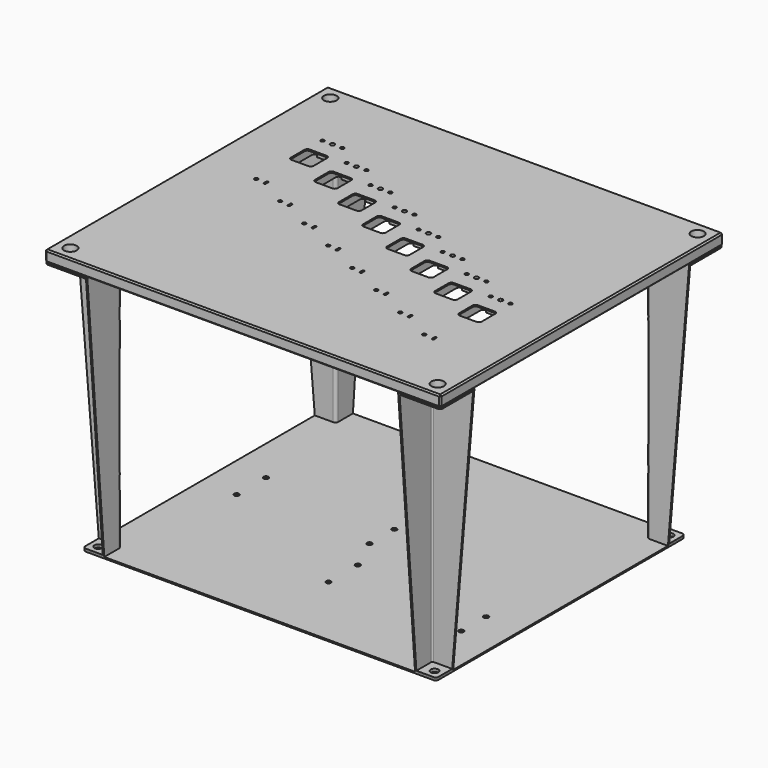
from build123d import *

# Parameters (mm, degrees)
F0_W              = 280
F0_H              = 250
F0_R              = 1.25
F0_R_2            = 1.525
F1_DEPTH          = 8
F2_W              = 30
F2_H              = 30
F4_W              = 15
F4_H              = 15
F9_T              = -1
F9_2_T            = -1
F9_3_T            = -1
F9_4_T            = -1
F10_W             = 250
F10_H             = 220
F11_DEPTH         = 1
F12_R             = 2.75
F13_DEPTH         = 25
F15_D             = 5.5
F15_DEPTH         = 20
F15_CBORE_D       = 9
F15_CBORE_DEPTH   = 5.5
F15_TIP           = 1.6523667023
F15_2_D           = 5.5
F15_2_DEPTH       = 20
F15_2_CBORE_D     = 9
F15_2_CBORE_DEPTH = 5.5
F15_2_TIP         = 1.6523667023
F15_3_D           = 5.5
F15_3_DEPTH       = 20
F15_3_CBORE_D     = 9
F15_3_CBORE_DEPTH = 5.5
F15_3_TIP         = 1.6523667023
F15_4_D           = 5.5
F15_4_DEPTH       = 20
F15_4_CBORE_D     = 9
F15_4_CBORE_DEPTH = 5.5
F15_4_TIP         = 1.6523667023
F15_5_D           = 5.5
F15_5_DEPTH       = 20
F15_5_CBORE_D     = 9
F15_5_CBORE_DEPTH = 5.5
F15_5_TIP         = 1.6523667023
F16_R             = 2
F16_2_R           = 2
F16_3_R           = 2
F16_4_R           = 2
F17_R             = 1
F17_2_R           = 1
F17_3_R           = 1
F17_4_R           = 1
F19_DEPTH         = 7
F21_DEPTH         = 5
F22_R             = 1.75
F23_DEPTH         = 1.001
F24_SIZE          = 1
F25_R             = 2
F25_2_R           = 2
F25_3_R           = 2
F25_4_R           = 2
F25_5_R           = 2


with BuildPart() as f1:
    # F0 (on Top) → F1 (new body)
    with BuildSketch(Plane.XY):
        Rectangle(F0_W, F0_H)
        with Locations((-47.5, -11.22)):
            Circle(F0_R, mode=Mode.SUBTRACT)
        with BuildLine():
            Line((-41.265, -12.22), (-41.265, -10.22))
            ThreePointArc((-41.265, -10.22), (-40.5, -9.455), (-39.735, -10.22))
            Line((-39.735, -10.22), (-39.735, -12.22))
            ThreePointArc((-39.735, -12.22), (-40.5, -12.985), (-41.265, -12.22))
        make_face(mode=Mode.SUBTRACT)
        with Locations((-20.5, -23.72)):
            Circle(F0_R, mode=Mode.SUBTRACT)
        with BuildLine():
            Line((-12.735, -22.72), (-12.735, -24.72))
            ThreePointArc((-12.735, -24.72), (-13.5, -25.485), (-14.265, -24.72))
            Line((-14.265, -24.72), (-14.265, -22.72))
            ThreePointArc((-14.265, -22.72), (-13.5, -21.955), (-12.735, -22.72))
        make_face(mode=Mode.SUBTRACT)
        with Locations((87.5, -73.72)):
            Circle(F0_R, mode=Mode.SUBTRACT)
        with BuildLine():
            Line((95.265, -72.72), (95.265, -74.72))
            ThreePointArc((95.265, -74.72), (94.5, -75.485), (93.735, -74.72))
            Line((93.735, -74.72), (93.735, -72.72))
            ThreePointArc((93.735, -72.72), (94.5, -71.955), (95.265, -72.72))
        make_face(mode=Mode.SUBTRACT)
        with Locations((33.5, -48.72)):
            Circle(F0_R, mode=Mode.SUBTRACT)
        with Locations((6.5, -36.22)):
            Circle(F0_R, mode=Mode.SUBTRACT)
        with BuildLine():
            Line((14.265, -35.22), (14.265, -37.22))
            ThreePointArc((14.265, -37.22), (13.5, -37.985), (12.735, -37.22))
            Line((12.735, -37.22), (12.735, -35.22))
            ThreePointArc((12.735, -35.22), (13.5, -34.455), (14.265, -35.22))
        make_face(mode=Mode.SUBTRACT)
        with BuildLine():
            Line((41.265, -47.72), (41.265, -49.72))
            ThreePointArc((41.265, -49.72), (40.5, -50.485), (39.735, -49.72))
            Line((39.735, -49.72), (39.735, -47.72))
            ThreePointArc((39.735, -47.72), (40.5, -46.955), (41.265, -47.72))
        make_face(mode=Mode.SUBTRACT)
        with Locations((60.5, -61.22)):
            Circle(F0_R, mode=Mode.SUBTRACT)
        with BuildLine():
            Line((68.265, -60.22), (68.265, -62.22))
            ThreePointArc((68.265, -62.22), (67.5, -62.985), (66.735, -62.22))
            Line((66.735, -62.22), (66.735, -60.22))
            ThreePointArc((66.735, -60.22), (67.5, -59.455), (68.265, -60.22))
        make_face(mode=Mode.SUBTRACT)
        with BuildLine():
            Line((73.5, -31.2), (61.5, -31.2))
            ThreePointArc((61.5, -31.2), (60.0857864376, -30.6142135624), (59.5, -29.2))
            Line((59.5, -29.2), (59.5, -17.2))
            ThreePointArc((59.5, -17.2), (60.0857864376, -15.7857864376), (61.5, -15.2))
            Line((61.5, -15.2), (73.5, -15.2))
            ThreePointArc((73.5, -15.2), (74.9142135624, -15.7857864376), (75.5, -17.2))
            Line((75.5, -17.2), (75.5, -29.2))
            ThreePointArc((75.5, -29.2), (74.9142135624, -30.6142135624), (73.5, -31.2))
        make_face(mode=Mode.SUBTRACT)
        with BuildLine():
            Line((46.5, -18.7), (34.5, -18.7))
            ThreePointArc((34.5, -18.7), (33.0857864376, -18.1142135624), (32.5, -16.7))
            Line((32.5, -16.7), (32.5, -4.7))
            ThreePointArc((32.5, -4.7), (33.0857864376, -3.2857864376), (34.5, -2.7))
            Line((34.5, -2.7), (46.5, -2.7))
            ThreePointArc((46.5, -2.7), (47.9142135624, -3.2857864376), (48.5, -4.7))
            Line((48.5, -4.7), (48.5, -16.7))
            ThreePointArc((48.5, -16.7), (47.9142135624, -18.1142135624), (46.5, -18.7))
        make_face(mode=Mode.SUBTRACT)
        with Locations((60.5, -2.5)):
            Circle(F0_R, mode=Mode.SUBTRACT)
        with Locations((67.5, -2.5)):
            Circle(F0_R_2, mode=Mode.SUBTRACT)
        with BuildLine():
            Line((100.5, -43.7), (88.5, -43.7))
            ThreePointArc((88.5, -43.7), (87.0857864376, -43.1142135624), (86.5, -41.7))
            Line((86.5, -41.7), (86.5, -29.7))
            ThreePointArc((86.5, -29.7), (87.0857864376, -28.2857864376), (88.5, -27.7))
            Line((88.5, -27.7), (100.5, -27.7))
            ThreePointArc((100.5, -27.7), (101.9142135624, -28.2857864376), (102.5, -29.7))
            Line((102.5, -29.7), (102.5, -41.7))
            ThreePointArc((102.5, -41.7), (101.9142135624, -43.1142135624), (100.5, -43.7))
        make_face(mode=Mode.SUBTRACT)
        with Locations((74.5, -2.5)):
            Circle(F0_R, mode=Mode.SUBTRACT)
        with Locations((87.5, -15)):
            Circle(F0_R, mode=Mode.SUBTRACT)
        with Locations((94.5, -15)):
            Circle(F0_R_2, mode=Mode.SUBTRACT)
        with Locations((101.5, -15)):
            Circle(F0_R, mode=Mode.SUBTRACT)
        with Locations((-101.5, 13.78)):
            Circle(F0_R, mode=Mode.SUBTRACT)
        with BuildLine():
            Line((-93.735, 14.78), (-93.735, 12.78))
            ThreePointArc((-93.735, 12.78), (-94.5, 12.015), (-95.265, 12.78))
            Line((-95.265, 12.78), (-95.265, 14.78))
            ThreePointArc((-95.265, 14.78), (-94.5, 15.545), (-93.735, 14.78))
        make_face(mode=Mode.SUBTRACT)
        with Locations((-74.5, 1.28)):
            Circle(F0_R, mode=Mode.SUBTRACT)
        with BuildLine():
            Line((-88.5, 43.8), (-100.5, 43.8))
            ThreePointArc((-100.5, 43.8), (-101.9142135624, 44.3857864376), (-102.5, 45.8))
            Line((-102.5, 45.8), (-102.5, 57.8))
            ThreePointArc((-102.5, 57.8), (-101.9142135624, 59.2142135624), (-100.5, 59.8))
            Line((-100.5, 59.8), (-88.5, 59.8))
            ThreePointArc((-88.5, 59.8), (-87.0857864376, 59.2142135624), (-86.5, 57.8))
            Line((-86.5, 57.8), (-86.5, 45.8))
            ThreePointArc((-86.5, 45.8), (-87.0857864376, 44.3857864376), (-88.5, 43.8))
        make_face(mode=Mode.SUBTRACT)
        with Locations((-74.5, 60)):
            Circle(F0_R, mode=Mode.SUBTRACT)
        with BuildLine():
            Line((-66.735, 2.28), (-66.735, 0.28))
            ThreePointArc((-66.735, 0.28), (-67.5, -0.485), (-68.265, 0.28))
            Line((-68.265, 0.28), (-68.265, 2.28))
            ThreePointArc((-68.265, 2.28), (-67.5, 3.045), (-66.735, 2.28))
        make_face(mode=Mode.SUBTRACT)
        with BuildLine():
            ThreePointArc((-48.5, 32.8), (-47.9142135624, 34.2142135624), (-46.5, 34.8))
            Line((-46.5, 34.8), (-34.5, 34.8))
            ThreePointArc((-34.5, 34.8), (-33.0857864376, 34.2142135624), (-32.5, 32.8))
            Line((-32.5, 32.8), (-32.5, 20.8))
            ThreePointArc((-32.5, 20.8), (-33.0857864376, 19.3857864376), (-34.5, 18.8))
            Line((-34.5, 18.8), (-46.5, 18.8))
            ThreePointArc((-46.5, 18.8), (-47.9142135624, 19.3857864376), (-48.5, 20.8))
            Line((-48.5, 20.8), (-48.5, 32.8))
        make_face(mode=Mode.SUBTRACT)
        with BuildLine():
            Line((-7.5, 6.3), (-19.5, 6.3))
            ThreePointArc((-19.5, 6.3), (-20.9142135624, 6.8857864376), (-21.5, 8.3))
            Line((-21.5, 8.3), (-21.5, 20.3))
            ThreePointArc((-21.5, 20.3), (-20.9142135624, 21.7142135624), (-19.5, 22.3))
            Line((-19.5, 22.3), (-7.5, 22.3))
            ThreePointArc((-7.5, 22.3), (-6.0857864376, 21.7142135624), (-5.5, 20.3))
            Line((-5.5, 20.3), (-5.5, 8.3))
            ThreePointArc((-5.5, 8.3), (-6.0857864376, 6.8857864376), (-7.5, 6.3))
        make_face(mode=Mode.SUBTRACT)
        with BuildLine():
            Line((-61.5, 31.3), (-73.5, 31.3))
            ThreePointArc((-73.5, 31.3), (-74.9142135624, 31.8857864376), (-75.5, 33.3))
            Line((-75.5, 33.3), (-75.5, 45.3))
            ThreePointArc((-75.5, 45.3), (-74.9142135624, 46.7142135624), (-73.5, 47.3))
            Line((-73.5, 47.3), (-61.5, 47.3))
            ThreePointArc((-61.5, 47.3), (-60.0857864376, 46.7142135624), (-59.5, 45.3))
            Line((-59.5, 45.3), (-59.5, 33.3))
            ThreePointArc((-59.5, 33.3), (-60.0857864376, 31.8857864376), (-61.5, 31.3))
        make_face(mode=Mode.SUBTRACT)
        with Locations((-67.5, 60)):
            Circle(F0_R_2, mode=Mode.SUBTRACT)
        with Locations((-60.5, 60)):
            Circle(F0_R, mode=Mode.SUBTRACT)
        with Locations((-47.5, 47.5)):
            Circle(F0_R, mode=Mode.SUBTRACT)
        with Locations((-40.5, 47.5)):
            Circle(F0_R_2, mode=Mode.SUBTRACT)
        with Locations((-20.5, 35)):
            Circle(F0_R, mode=Mode.SUBTRACT)
        with Locations((-13.5, 35)):
            Circle(F0_R_2, mode=Mode.SUBTRACT)
        with Locations((-6.5, 35)):
            Circle(F0_R, mode=Mode.SUBTRACT)
        with Locations((-33.5, 47.5)):
            Circle(F0_R, mode=Mode.SUBTRACT)
        with Locations((-101.5, 72.5)):
            Circle(F0_R, mode=Mode.SUBTRACT)
        with Locations((-94.5, 72.5)):
            Circle(F0_R_2, mode=Mode.SUBTRACT)
        with Locations((-87.5, 72.5)):
            Circle(F0_R, mode=Mode.SUBTRACT)
        with BuildLine():
            Line((19.5, -6.2), (7.5, -6.2))
            ThreePointArc((7.5, -6.2), (6.0857864376, -5.6142135624), (5.5, -4.2))
            Line((5.5, -4.2), (5.5, 7.8))
            ThreePointArc((5.5, 7.8), (6.0857864376, 9.2142135624), (7.5, 9.8))
            Line((7.5, 9.8), (19.5, 9.8))
            ThreePointArc((19.5, 9.8), (20.9142135624, 9.2142135624), (21.5, 7.8))
            Line((21.5, 7.8), (21.5, -4.2))
            ThreePointArc((21.5, -4.2), (20.9142135624, -5.6142135624), (19.5, -6.2))
        make_face(mode=Mode.SUBTRACT)
        with Locations((33.5, 10)):
            Circle(F0_R, mode=Mode.SUBTRACT)
        with Locations((6.5, 22.5)):
            Circle(F0_R, mode=Mode.SUBTRACT)
        with Locations((13.5, 22.5)):
            Circle(F0_R_2, mode=Mode.SUBTRACT)
        with Locations((20.5, 22.5)):
            Circle(F0_R, mode=Mode.SUBTRACT)
        with Locations((40.5, 10)):
            Circle(F0_R_2, mode=Mode.SUBTRACT)
        with Locations((47.5, 10)):
            Circle(F0_R, mode=Mode.SUBTRACT)
    extrude(amount=F1_DEPTH)

    # F15
    with Locations(Plane.XY.offset(8)):
        with Locations((130, 115), (130, -115), (-130, -115), (-130, 115)):
            CounterBoreHole(F15_D / 2, F15_CBORE_D / 2, F15_CBORE_DEPTH, depth=F15_DEPTH)
            with Locations((0, 0, -(F15_DEPTH + F15_TIP / 2))):  # 118° drill point
                Cone(0, F15_D / 2, F15_TIP, mode=Mode.SUBTRACT)

    # F18 (on face) → F19 (cut)
    with BuildSketch(Plane(origin=(0, 0, 0), x_dir=(1, 0, 0), z_dir=(0, 0, -1))):
        with BuildLine():
            Line((86, 24.7), (103, 24.7))
            ThreePointArc((103, 24.7), (104.4142135624, 25.2857864376), (105, 26.7))
            Line((105, 26.7), (105, 43.7))
            ThreePointArc((105, 43.7), (104.4142135624, 45.1142135624), (103, 45.7))
            Line((103, 45.7), (86, 45.7))
            ThreePointArc((86, 45.7), (84.5857864376, 45.1142135624), (84, 43.7))
            Line((84, 43.7), (84, 26.7))
            ThreePointArc((84, 26.7), (84.5857864376, 25.2857864376), (86, 24.7))
        make_face()
        with BuildLine():
            ThreePointArc((76, 12.2), (77.4142135624, 12.7857864376), (78, 14.2))
            Line((78, 14.2), (78, 31.2))
            ThreePointArc((78, 31.2), (77.4142135624, 32.6142135624), (76, 33.2))
            Line((76, 33.2), (59, 33.2))
            ThreePointArc((59, 33.2), (57.5857864376, 32.6142135624), (57, 31.2))
            Line((57, 31.2), (57, 14.2))
            ThreePointArc((57, 14.2), (57.5857864376, 12.7857864376), (59, 12.2))
            Line((59, 12.2), (76, 12.2))
        make_face()
        with BuildLine():
            ThreePointArc((49, -0.3), (50.4142135624, 0.2857864376), (51, 1.7))
            Line((51, 1.7), (51, 18.7))
            ThreePointArc((51, 18.7), (50.4142135624, 20.1142135624), (49, 20.7))
            Line((49, 20.7), (32, 20.7))
            ThreePointArc((32, 20.7), (30.5857864376, 20.1142135624), (30, 18.7))
            Line((30, 18.7), (30, 1.7))
            ThreePointArc((30, 1.7), (30.5857864376, 0.2857864376), (32, -0.3))
            Line((32, -0.3), (49, -0.3))
        make_face()
        with BuildLine():
            ThreePointArc((22, -12.8), (23.4142135624, -12.2142135624), (24, -10.8))
            Line((24, -10.8), (24, 6.2))
            ThreePointArc((24, 6.2), (23.4142135624, 7.6142135624), (22, 8.2))
            Line((22, 8.2), (5, 8.2))
            ThreePointArc((5, 8.2), (3.5857864376, 7.6142135624), (3, 6.2))
            Line((3, 6.2), (3, -10.8))
            ThreePointArc((3, -10.8), (3.5857864376, -12.2142135624), (5, -12.8))
            Line((5, -12.8), (22, -12.8))
        make_face()
        with BuildLine():
            ThreePointArc((-5, -25.3), (-3.5857864376, -24.7142135624), (-3, -23.3))
            Line((-3, -23.3), (-3, -6.3))
            ThreePointArc((-3, -6.3), (-3.5857864376, -4.8857864376), (-5, -4.3))
            Line((-5, -4.3), (-22, -4.3))
            ThreePointArc((-22, -4.3), (-23.4142135624, -4.8857864376), (-24, -6.3))
            Line((-24, -6.3), (-24, -23.3))
            ThreePointArc((-24, -23.3), (-23.4142135624, -24.7142135624), (-22, -25.3))
            Line((-22, -25.3), (-5, -25.3))
        make_face()
        with BuildLine():
            ThreePointArc((-32, -37.8), (-30.5857864376, -37.2142135624), (-30, -35.8))
            Line((-30, -35.8), (-30, -18.8))
            ThreePointArc((-30, -18.8), (-30.5857864376, -17.3857864376), (-32, -16.8))
            Line((-32, -16.8), (-49, -16.8))
            ThreePointArc((-49, -16.8), (-50.4142135624, -17.3857864376), (-51, -18.8))
            Line((-51, -18.8), (-51, -35.8))
            ThreePointArc((-51, -35.8), (-50.4142135624, -37.2142135624), (-49, -37.8))
            Line((-49, -37.8), (-32, -37.8))
        make_face()
        with BuildLine():
            ThreePointArc((-59, -50.3), (-57.5857864376, -49.7142135624), (-57, -48.3))
            Line((-57, -48.3), (-57, -31.3))
            ThreePointArc((-57, -31.3), (-57.5857864376, -29.8857864376), (-59, -29.3))
            Line((-59, -29.3), (-76, -29.3))
            ThreePointArc((-76, -29.3), (-77.4142135624, -29.8857864376), (-78, -31.3))
            Line((-78, -31.3), (-78, -48.3))
            ThreePointArc((-78, -48.3), (-77.4142135624, -49.7142135624), (-76, -50.3))
            Line((-76, -50.3), (-59, -50.3))
        make_face()
        with BuildLine():
            ThreePointArc((-86, -62.8), (-84.5857864376, -62.2142135624), (-84, -60.8))
            Line((-84, -60.8), (-84, -43.8))
            ThreePointArc((-84, -43.8), (-84.5857864376, -42.3857864376), (-86, -41.8))
            Line((-86, -41.8), (-103, -41.8))
            ThreePointArc((-103, -41.8), (-104.4142135624, -42.3857864376), (-105, -43.8))
            Line((-105, -43.8), (-105, -60.8))
            ThreePointArc((-105, -60.8), (-104.4142135624, -62.2142135624), (-103, -62.8))
            Line((-103, -62.8), (-86, -62.8))
        make_face()
    extrude(amount=-F19_DEPTH, mode=Mode.SUBTRACT)

    # F20 (on face) → F21 (cut)
    with BuildSketch(Plane(origin=(0, 0, 0), x_dir=(1, 0, 0), z_dir=(0, 0, -1))):
        with BuildLine():
            Line((105, 19.7), (105, 26.7))
            Line((105, 26.7), (84, 26.7))
            Line((84, 26.7), (84, 19.7))
            ThreePointArc((84, 19.7), (86, 17.7), (88, 19.7))
            Line((88, 19.7), (101, 19.7))
            ThreePointArc((101, 19.7), (103, 17.7), (105, 19.7))
        make_face()
        with BuildLine():
            Line((61, 7.3), (74, 7.3))
            ThreePointArc((74, 7.3), (76, 5.3), (78, 7.3))
            Line((78, 7.3), (78, 14.2))
            Line((78, 14.2), (57, 14.2))
            Line((57, 14.2), (57, 7.3))
            ThreePointArc((57, 7.3), (59, 5.3), (61, 7.3))
        make_face()
        with BuildLine():
            Line((51, -5.1), (51, 1.7))
            Line((51, 1.7), (30, 1.7))
            Line((30, 1.7), (30, -5.1))
            ThreePointArc((30, -5.1), (32, -7.1), (34, -5.1))
            Line((34, -5.1), (47, -5.1))
            ThreePointArc((47, -5.1), (49, -7.1), (51, -5.1))
        make_face()
        with BuildLine():
            Line((24, -17.5), (24, -10.8))
            Line((24, -10.8), (3, -10.8))
            Line((3, -10.8), (3, -17.5))
            ThreePointArc((3, -17.5), (5, -19.5), (7, -17.5))
            Line((7, -17.5), (20, -17.5))
            ThreePointArc((20, -17.5), (22, -19.5), (24, -17.5))
        make_face()
        with BuildLine():
            Line((-3, -29.9), (-3, -23.3))
            Line((-3, -23.3), (-24, -23.3))
            Line((-24, -23.3), (-24, -29.9))
            ThreePointArc((-24, -29.9), (-22, -31.9), (-20, -29.9))
            Line((-20, -29.9), (-7, -29.9))
            ThreePointArc((-7, -29.9), (-5, -31.9), (-3, -29.9))
        make_face()
        with BuildLine():
            Line((-30, -42.3), (-30, -35.8))
            Line((-30, -35.8), (-51, -35.8))
            Line((-51, -35.8), (-51, -42.3))
            ThreePointArc((-51, -42.3), (-49, -44.3), (-47, -42.3))
            Line((-47, -42.3), (-34, -42.3))
            ThreePointArc((-34, -42.3), (-32, -44.3), (-30, -42.3))
        make_face()
        with BuildLine():
            Line((-57, -54.7), (-57, -48.3))
            Line((-57, -48.3), (-78, -48.3))
            Line((-78, -48.3), (-78, -54.7))
            ThreePointArc((-78, -54.7), (-76, -56.7), (-74, -54.7))
            Line((-74, -54.7), (-61, -54.7))
            ThreePointArc((-61, -54.7), (-59, -56.7), (-57, -54.7))
        make_face()
        with BuildLine():
            Line((-84, -67.1), (-84, -60.8))
            Line((-84, -60.8), (-105, -60.8))
            Line((-105, -60.8), (-105, -67.1))
            ThreePointArc((-105, -67.1), (-103, -69.1), (-101, -67.1))
            Line((-101, -67.1), (-88, -67.1))
            ThreePointArc((-88, -67.1), (-86, -69.1), (-84, -67.1))
        make_face()
    extrude(amount=-F21_DEPTH, mode=Mode.SUBTRACT)

    # F24
    f24_edges = [f1.edges().sort_by_distance(p)[0] for p in [
        (0, 125, 8),
        (-140, 0, 8),
        (-140, 125, 4),
        (0, 125, 0),
        (-140, 0, 0),
        (140, -125, 4),
        (140, 0, 8),
        (0, -125, 8),
        (140, 0, 0),
        (140, 125, 4),
        (-140, -125, 4),
        (0, -125, 0),
    ]]
    chamfer(f24_edges, length=F24_SIZE)


with BuildPart() as f5:
    # F2 (on face) → F5 section 0
    with BuildSketch(Plane(origin=(0, 0, 0), x_dir=(1, 0, 0), z_dir=(0, 0, -1))):
        with Locations((-125, 110)):
            Rectangle(F2_W, F2_H)
    # F4 (on offset) → F5 section 1
    with BuildSketch(Plane(origin=(0, 0, -180), x_dir=(1, 0, 0), z_dir=(0, 0, -1))):
        with Locations((-117.5, 102.5)):
            Rectangle(F4_W, F4_H)
    loft()

    # F9
    f9_openings = [f5.faces().sort_by_distance(p)[0] for p in [
        (-133.333333, -106.666667, -80),
        (-121.666667, -118.333333, -80),
    ]]
    offset(amount=F9_T, openings=f9_openings, kind=Kind.INTERSECTION)


with BuildPart() as f6:
    # F2 (on face) → F6 section 0
    with BuildSketch(Plane(origin=(0, 0, 0), x_dir=(1, 0, 0), z_dir=(0, 0, -1))):
        with Locations((125, 110)):
            Rectangle(F2_W, F2_H)
    # F4 (on offset) → F6 section 1
    with BuildSketch(Plane(origin=(0, 0, -180), x_dir=(1, 0, 0), z_dir=(0, 0, -1))):
        with Locations((117.5, 102.5)):
            Rectangle(F4_W, F4_H)
    loft()

    # F9#2
    f9_2_openings = [f6.faces().sort_by_distance(p)[0] for p in [
        (133.333333, -106.666667, -80),
        (121.666667, -118.333333, -80),
    ]]
    offset(amount=F9_2_T, openings=f9_2_openings, kind=Kind.INTERSECTION)


with BuildPart() as f7:
    # F2 (on face) → F7 section 0
    with BuildSketch(Plane(origin=(0, 0, 0), x_dir=(1, 0, 0), z_dir=(0, 0, -1))):
        with Locations((-125, -110)):
            Rectangle(F2_W, F2_H)
    # F4 (on offset) → F7 section 1
    with BuildSketch(Plane(origin=(0, 0, -180), x_dir=(1, 0, 0), z_dir=(0, 0, -1))):
        with Locations((-117.5, -102.5)):
            Rectangle(F4_W, F4_H)
    loft()

    # F9#4
    f9_4_openings = [f7.faces().sort_by_distance(p)[0] for p in [
        (-121.666667, 118.333333, -80),
        (-133.333333, 106.666667, -80),
    ]]
    offset(amount=F9_4_T, openings=f9_4_openings, kind=Kind.INTERSECTION)


with BuildPart() as f8:
    # F2 (on face) → F8 section 0
    with BuildSketch(Plane(origin=(0, 0, 0), x_dir=(1, 0, 0), z_dir=(0, 0, -1))):
        with Locations((125, -110)):
            Rectangle(F2_W, F2_H)
    # F4 (on offset) → F8 section 1
    with BuildSketch(Plane(origin=(0, 0, -180), x_dir=(1, 0, 0), z_dir=(0, 0, -1))):
        with Locations((117.5, -102.5)):
            Rectangle(F4_W, F4_H)
    loft()

    # F9#3
    f9_3_openings = [f8.faces().sort_by_distance(p)[0] for p in [
        (121.666667, 118.333333, -80),
        (133.333333, 106.666667, -80),
    ]]
    offset(amount=F9_3_T, openings=f9_3_openings, kind=Kind.INTERSECTION)


with BuildPart() as f11:
    # F10 (on offset) → F11 (new body)
    with BuildSketch(Plane(origin=(0, 0, -180), x_dir=(1, 0, 0), z_dir=(0, 0, -1))):
        Rectangle(F10_W, F10_H)
    extrude(amount=F11_DEPTH)


with BuildPart() as f13_tool:
    # F12 (on face) → F13 (new body)
    with BuildSketch(Plane(origin=(0, 0, -181), x_dir=(1, 0, 0), z_dir=(0, 0, -1))):
        with Locations((-119.0833333333, 104)):
            Circle(F12_R)
        with Locations((-119.0833333333, -104)):
            Circle(F12_R)
        with Locations((119, -104)):
            Circle(F12_R)
        with Locations((119, 104)):
            Circle(F12_R)
    extrude(amount=-F13_DEPTH)


with BuildPart() as f5_1:
    add(f5.part)

    # F13: cut by f13_tool
    add(f13_tool.part, mode=Mode.SUBTRACT)

    # F15#2
    with Locations(Plane.XY.offset(8)):
        with Locations((130, 115), (130, -115), (-130, -115), (-130, 115)):
            CounterBoreHole(F15_2_D / 2, F15_2_CBORE_D / 2, F15_2_CBORE_DEPTH, depth=F15_2_DEPTH)
            with Locations((0, 0, -(F15_2_DEPTH + F15_2_TIP / 2))):  # 118° drill point
                Cone(0, F15_2_D / 2, F15_2_TIP, mode=Mode.SUBTRACT)

    # F16
    f16_edges = [f5_1.edges().sort_by_distance(p)[0] for p in [
        (-110, -95, -90),
    ]]
    fillet(f16_edges, radius=F16_R)

    # F17
    f17_edges = [f5_1.edges().sort_by_distance(p)[0] for p in [
        (-111, -96, -90),
    ]]
    fillet(f17_edges, radius=F17_R)

    # F25
    f25_edges = [f5_1.edges().sort_by_distance(p)[0] for p in [
        (-125.041667, -110.041667, -179.5),
        (-139.958333, -124.958333, -0.5),
    ]]
    fillet(f25_edges, radius=F25_R)


with BuildPart() as f6_1:
    add(f6.part)

    # F13: cut by f13_tool
    add(f13_tool.part, mode=Mode.SUBTRACT)

    # F15#3
    with Locations(Plane.XY.offset(8)):
        with Locations((130, 115), (130, -115), (-130, -115), (-130, 115)):
            CounterBoreHole(F15_3_D / 2, F15_3_CBORE_D / 2, F15_3_CBORE_DEPTH, depth=F15_3_DEPTH)
            with Locations((0, 0, -(F15_3_DEPTH + F15_3_TIP / 2))):  # 118° drill point
                Cone(0, F15_3_D / 2, F15_3_TIP, mode=Mode.SUBTRACT)

    # F16#2
    f16_2_edges = [f6_1.edges().sort_by_distance(p)[0] for p in [
        (110, -95, -90),
    ]]
    fillet(f16_2_edges, radius=F16_2_R)

    # F17#2
    f17_2_edges = [f6_1.edges().sort_by_distance(p)[0] for p in [
        (111, -96, -90),
    ]]
    fillet(f17_2_edges, radius=F17_2_R)

    # F25#2
    f25_2_edges = [f6_1.edges().sort_by_distance(p)[0] for p in [
        (139.958333, -124.958333, -0.5),
        (125.041667, -110.041667, -179.5),
    ]]
    fillet(f25_2_edges, radius=F25_2_R)


with BuildPart() as f7_1:
    add(f7.part)

    # F13: cut by f13_tool
    add(f13_tool.part, mode=Mode.SUBTRACT)

    # F15#4
    with Locations(Plane.XY.offset(8)):
        with Locations((130, 115), (130, -115), (-130, -115), (-130, 115)):
            CounterBoreHole(F15_4_D / 2, F15_4_CBORE_D / 2, F15_4_CBORE_DEPTH, depth=F15_4_DEPTH)
            with Locations((0, 0, -(F15_4_DEPTH + F15_4_TIP / 2))):  # 118° drill point
                Cone(0, F15_4_D / 2, F15_4_TIP, mode=Mode.SUBTRACT)

    # F16#3
    f16_3_edges = [f7_1.edges().sort_by_distance(p)[0] for p in [
        (-110, 95, -90),
    ]]
    fillet(f16_3_edges, radius=F16_3_R)

    # F17#3
    f17_3_edges = [f7_1.edges().sort_by_distance(p)[0] for p in [
        (-111, 96, -90),
    ]]
    fillet(f17_3_edges, radius=F17_3_R)

    # F25#3
    f25_3_edges = [f7_1.edges().sort_by_distance(p)[0] for p in [
        (-139.958333, 124.958333, -0.5),
        (-125.041667, 110.041667, -179.5),
    ]]
    fillet(f25_3_edges, radius=F25_3_R)


with BuildPart() as f8_1:
    add(f8.part)

    # F13: cut by f13_tool
    add(f13_tool.part, mode=Mode.SUBTRACT)

    # F15#5
    with Locations(Plane.XY.offset(8)):
        with Locations((130, 115), (130, -115), (-130, -115), (-130, 115)):
            CounterBoreHole(F15_5_D / 2, F15_5_CBORE_D / 2, F15_5_CBORE_DEPTH, depth=F15_5_DEPTH)
            with Locations((0, 0, -(F15_5_DEPTH + F15_5_TIP / 2))):  # 118° drill point
                Cone(0, F15_5_D / 2, F15_5_TIP, mode=Mode.SUBTRACT)

    # F16#4
    f16_4_edges = [f8_1.edges().sort_by_distance(p)[0] for p in [
        (110, 95, -90),
    ]]
    fillet(f16_4_edges, radius=F16_4_R)

    # F17#4
    f17_4_edges = [f8_1.edges().sort_by_distance(p)[0] for p in [
        (111, 96, -90),
    ]]
    fillet(f17_4_edges, radius=F17_4_R)

    # F25#4
    f25_4_edges = [f8_1.edges().sort_by_distance(p)[0] for p in [
        (139.958333, 124.958333, -0.5),
        (125.041667, 110.041667, -179.5),
    ]]
    fillet(f25_4_edges, radius=F25_4_R)


with BuildPart() as f11_1:
    add(f11.part)

    # F13: cut by f13_tool
    add(f13_tool.part, mode=Mode.SUBTRACT)

    # F22 (on face) → F23 (cut, through all)
    with BuildSketch(Plane.XY.offset(-180)):
        with Locations((-99.5, 20)):
            Circle(F22_R)
        with Locations((-5.5, 16)):
            Circle(F22_R)
        with Locations((-99.5, -6)):
            Circle(F22_R)
        with Locations((-5.5, -6)):
            Circle(F22_R)
        with Locations((5.5, -30)):
            Circle(F22_R)
        with Locations((99.5, -34)):
            Circle(F22_R)
        with Locations((5.5, -56)):
            Circle(F22_R)
        with Locations((99.5, -56)):
            Circle(F22_R)
    extrude(amount=-F23_DEPTH, mode=Mode.SUBTRACT)

    # F25#5
    f25_5_edges = [f11_1.edges().sort_by_distance(p)[0] for p in [
        (-125, 110, -180.5),
        (125, 110, -180.5),
        (125, -110, -180.5),
        (-125, -110, -180.5),
    ]]
    fillet(f25_5_edges, radius=F25_5_R)


solid = Compound([f1.part, f5_1.part, f6_1.part, f7_1.part, f8_1.part, f11_1.part])
